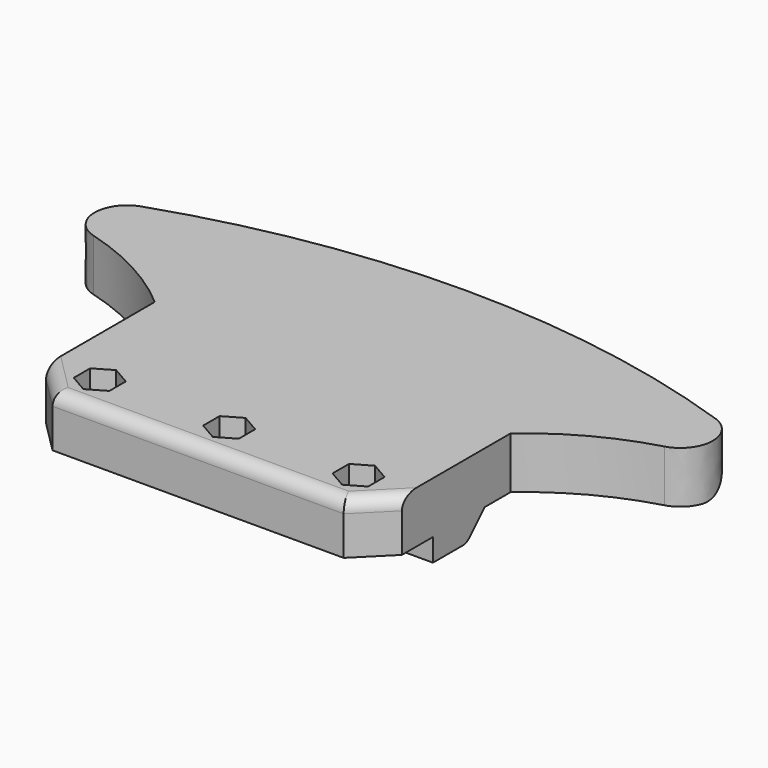
from build123d import *

# Parameters (mm, degrees)
F1_W        = 55
F1_H        = 5
F1_H_2      = 11
F2_DEPTH    = 8
F1_R        = 1.75
F3_DEPTH    = 4
F4_DEPTH    = 3.5
F5_T4_DEPTH = 55
F5_T6_DEPTH = 33.7168298797
F6_R        = 5
F7_R        = 2


# Not quite as in the source:
# - a fillet or chamfer that OpenCascade refuses, or shapes differently, is made with other operations: its cross-section is extruded or revolved along the edge and cut away or added
# - a feature names something its author has since deleted; it is built from what else it names


with BuildPart() as f2:
    # F1 (on Top) → F2 (new body)
    with BuildSketch(Plane.XY):
        with BuildLine():
            Line((-27.5, 10), (-27.5, 0))
            Line((-27.5, 0), (27.5, 0))
            Line((27.5, 0), (27.5, 10))
            ThreePointArc((27.5, 10), (45.1645357284, 19.1976835871), (65.078124404, 19.4843749404))
            ThreePointArc((65.078124404, 19.4843749404), (0, 35.8083822448), (-65.078124404, 19.4843749404))
            ThreePointArc((-65.078124404, 19.4843749404), (-45.1645357284, 19.1976835871), (-27.5, 10))
        make_face()
        with Locations((0, -2.5)):
            Rectangle(F1_W, F1_H)
        with Locations((0, -10.5)):
            Rectangle(F1_W, F1_H_2)
        Polygon((-20, -13.1754264805), (-22.75, -11.5877132403), (-22.75, -8.4122867597), (-20, -6.8245735195), (-17.25, -8.4122867597), (-17.25, -11.5877132403), align=None, mode=Mode.SUBTRACT)
        Polygon((0, -13.1754264805), (-2.75, -11.5877132403), (-2.75, -8.4122867597), (0, -6.8245735195), (2.75, -8.4122867597), (2.75, -11.5877132403), align=None, mode=Mode.SUBTRACT)
        Polygon((20, -13.1754264805), (17.25, -11.5877132403), (17.25, -8.4122867597), (20, -6.8245735195), (22.75, -8.4122867597), (22.75, -11.5877132403), align=None, mode=Mode.SUBTRACT)
    extrude(amount=F2_DEPTH)

    # F1 (on Top) → F3 (join)
    with BuildSketch(Plane.XY):
        Polygon((-22.75, -8.4122867597), (-22.75, -11.5877132403), (-20, -13.1754264805), (-17.25, -11.5877132403), (-17.25, -8.4122867597), (-20, -6.8245735195), align=None)
        with Locations((-20, -10)):
            Circle(F1_R, mode=Mode.SUBTRACT)
        Polygon((-2.75, -8.4122867597), (-2.75, -11.5877132403), (0, -13.1754264805), (2.75, -11.5877132403), (2.75, -8.4122867597), (0, -6.8245735195), align=None)
        with Locations((0, -10)):
            Circle(F1_R, mode=Mode.SUBTRACT)
        Polygon((17.25, -8.4122867597), (17.25, -11.5877132403), (20, -13.1754264805), (22.75, -11.5877132403), (22.75, -8.4122867597), (20, -6.8245735195), align=None)
        with Locations((20, -10)):
            Circle(F1_R, mode=Mode.SUBTRACT)
    extrude(amount=F3_DEPTH)

    # F1 (on Top) → F4 (join)
    with BuildSketch(Plane.XY):
        with Locations((0, -2.5)):
            Rectangle(F1_W, F1_H)
    extrude(amount=-F4_DEPTH)

    # F5: chamfer of 5 on 3 edges, made by hand


with BuildPart() as f5_tool2:
    # F5_s3 → F5_t4 (new body)
    with BuildSketch(Plane.YZ.offset(27.5)):
        Polygon((5, 0), (0, -5), (0, 0), align=None)
    extrude(amount=-F5_T4_DEPTH)

    split(bisect_by=Plane.XY.offset(-3.5), keep=Keep.TOP)


with BuildPart() as f2_1:
    add(f2.part)

    # F5_t1: union F5_tool2
    add(f5_tool2.part)

    # F5_s7 → F5_t6 (cut)
    with BuildSketch(Plane.XY.offset(-12.8584149398)):
        Polygon((-22.5, -16), (-27.5, -11), (-27.5, -16), align=None)
        Polygon((27.5, -11), (22.5, -16), (27.5, -16), align=None)
    extrude(amount=F5_T6_DEPTH, mode=Mode.SUBTRACT)

    # F6
    f6_edges = [f2_1.edges().sort_by_distance(p)[0] for p in [
        (0, 35.808382, 0),
        (-65.078124, 19.484375, 4),
        (65.078124, 19.484375, 4),
    ]]
    fillet(f6_edges, radius=F6_R)

    # F7
    f7_edges = [f2_1.edges().sort_by_distance(p)[0] for p in [
        (0, -16, 8),
        (-25, -13.5, 8),
        (25, -13.5, 8),
        (0, 1.5, -3.5),
    ]]
    fillet(f7_edges, radius=F7_R)


solid = f2_1.part
